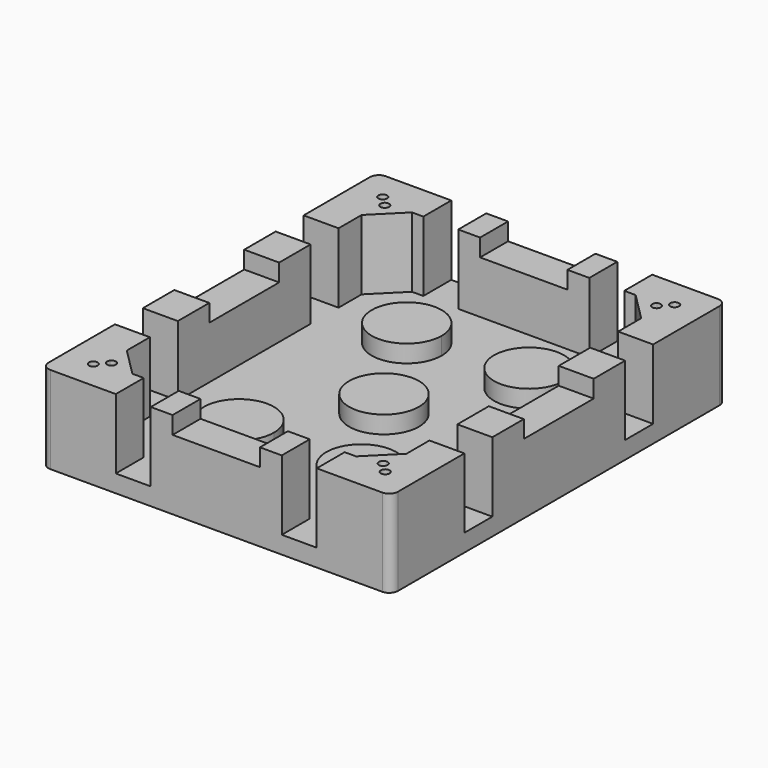
from build123d import *

# Parameters (mm, degrees)
F0_R     = 12.7
F0_R_2   = 1.5875
F0_W     = 6.35
F0_H     = 31.75
F0_W_2   = 31.75
F0_H_2   = 6.35
F0_H_3   = 14.2875
F0_H_4   = 12.7
F0_W_3   = 12.7
F0_W_4   = 7.9375
F1_DEPTH = 6.35
F2_DEPTH = 12.7
F3_DEPTH = 31.75
F4_DEPTH = 25.4


# Not quite as in the source:
# - a feature names something its author has since deleted; it is built from what else it names


with BuildPart() as f1:
    # F0 (on Top) → F1 (new body)
    with BuildSketch(Plane.XY):
        Polygon((-23.8125, 63.5), (-36.5125, 63.5), (-40.64, 63.5), (-50.8, 53.34), (-50.8, 42.8625), (-50.8, 30.1625), (-50.8, 15.875), (-50.8, -15.875), (-50.8, -30.1625), (-50.8, -42.8625), (-50.8, -53.34), (-40.64, -63.5), (-36.5125, -63.5), (-23.8125, -63.5), (-15.875, -63.5), (15.875, -63.5), (23.8125, -63.5), (36.5125, -63.5), (40.64, -63.5), (50.8, -53.34), (50.8, -42.8625), (50.8, -30.1625), (50.8, -15.875), (50.8, 15.875), (50.8, 30.1625), (50.8, 42.8625), (50.8, 53.34), (40.64, 63.5), (36.5125, 63.5), (23.8125, 63.5), (15.875, 63.5), (-15.875, 63.5), align=None)
        Polygon((-34.925, 38.1), (-34.925, 50.8), (-22.225, 50.8), (22.2250000973, 50.8), (34.925, 50.8), (34.925, 38.1), (34.925, -38.1), (34.925, -50.8), (22.2249999213, -50.8), (-22.225, -50.8), (-34.925, -50.8), (-34.925, -38.1), align=None, mode=Mode.SUBTRACT)
        with BuildLine():
            Line((22.2250000973, 50.8), (-22.225, 50.8))
            ThreePointArc((-22.225, 50.8), (-13.2447438789, 47.0802561211), (-9.525, 38.1))
            ThreePointArc((-9.525, 38.1), (-22.225, 25.4), (-34.925, 38.1))
            Line((-34.925, 38.1), (-34.925, -38.1))
            ThreePointArc((-34.925, -38.1), (-22.225, -25.4), (-9.525, -38.1))
            ThreePointArc((-9.525, -38.1), (-13.2447438789, -47.0802561211), (-22.225, -50.8))
            Line((-22.225, -50.8), (22.2249999213, -50.8))
            ThreePointArc((22.2249999213, -50.8), (13.2447439068, -29.1197438511), (34.925, -38.1))
            Line((34.925, -38.1), (34.925, 38.1))
            ThreePointArc((34.925, 38.1), (13.2447438445, 29.1197439133), (22.2250000973, 50.8))
        make_face()
        Circle(F0_R, mode=Mode.SUBTRACT)
        with BuildLine():
            ThreePointArc((34.925, 38.1), (31.2052561555, 47.0802560867), (22.2250000973, 50.8))
            ThreePointArc((22.2250000973, 50.8), (13.2447438445, 29.1197439133), (34.925, 38.1))
        make_face()
        Circle(F0_R)
        with BuildLine():
            ThreePointArc((-9.525, -38.1), (-22.225, -25.4), (-34.925, -38.1))
            ThreePointArc((-34.925, -38.1), (-31.2052561211, -47.0802561211), (-22.225, -50.8))
            ThreePointArc((-22.225, -50.8), (-13.2447438789, -47.0802561211), (-9.525, -38.1))
        make_face()
        with BuildLine():
            ThreePointArc((22.2249999213, -50.8), (31.2052560932, -47.0802561489), (34.925, -38.1))
            ThreePointArc((34.925, -38.1), (13.2447439068, -29.1197438511), (22.2249999213, -50.8))
        make_face()
        with BuildLine():
            ThreePointArc((-9.525, 38.1), (-13.2447438789, 47.0802561211), (-22.225, 50.8))
            ThreePointArc((-22.225, 50.8), (-31.2052561211, 47.0802561211), (-34.925, 38.1))
            ThreePointArc((-34.925, 38.1), (-22.225, 25.4), (-9.525, 38.1))
        make_face()
        with BuildLine():
            Line((-57.15, -42.8625), (-63.5, -42.8625))
            Line((-63.5, -42.8625), (-63.5, -73.025))
            ThreePointArc((-63.5, -73.025), (-62.5700640303, -75.2700640303), (-60.325, -76.2))
            Line((-60.325, -76.2), (-36.5125, -76.2))
            Line((-36.5125, -76.2), (-36.5125, -69.85))
            Line((-36.5125, -69.85), (-53.975, -69.85))
            ThreePointArc((-53.975, -69.85), (-56.2200640303, -68.9200640303), (-57.15, -66.675))
            Line((-57.15, -66.675), (-57.15, -42.8625))
        make_face()
        with BuildLine():
            Line((-36.5125, 76.2), (-60.325, 76.2))
            ThreePointArc((-60.325, 76.2), (-62.5700640303, 75.2700640303), (-63.5, 73.025))
            Line((-63.5, 73.025), (-63.5, 42.8625))
            Line((-63.5, 42.8625), (-57.15, 42.8625))
            Line((-57.15, 42.8625), (-57.15, 66.675))
            ThreePointArc((-57.15, 66.675), (-56.2200640303, 68.9200640303), (-53.975, 69.85))
            Line((-53.975, 69.85), (-36.5125, 69.85))
            Line((-36.5125, 69.85), (-36.5125, 76.2))
        make_face()
        with BuildLine():
            Line((60.325, 76.2), (36.5125, 76.2))
            Line((36.5125, 76.2), (36.5125, 69.85))
            Line((36.5125, 69.85), (53.975, 69.85))
            ThreePointArc((53.975, 69.85), (56.2200640303, 68.9200640303), (57.15, 66.675))
            Line((57.15, 66.675), (57.15, 42.8625))
            Line((57.15, 42.8625), (63.5, 42.8625))
            Line((63.5, 42.8625), (63.5, 73.025))
            ThreePointArc((63.5, 73.025), (62.5700640303, 75.2700640303), (60.325, 76.2))
        make_face()
        with BuildLine():
            Line((63.5, -73.025), (63.5, -42.8625))
            Line((63.5, -42.8625), (57.15, -42.8625))
            Line((57.15, -42.8625), (57.15, -66.675))
            ThreePointArc((57.15, -66.675), (56.2200640303, -68.9200640303), (53.975, -69.85))
            Line((53.975, -69.85), (36.5125, -69.85))
            Line((36.5125, -69.85), (36.5125, -76.2))
            Line((36.5125, -76.2), (60.325, -76.2))
            ThreePointArc((60.325, -76.2), (62.5700640303, -75.2700640303), (63.5, -73.025))
        make_face()
        with BuildLine():
            Line((-50.8, -42.8625), (-57.15, -42.8625))
            Line((-57.15, -42.8625), (-57.15, -66.675))
            ThreePointArc((-57.15, -66.675), (-56.2200640303, -68.9200640303), (-53.975, -69.85))
            Line((-53.975, -69.85), (-36.5125, -69.85))
            Line((-36.5125, -69.85), (-36.5125, -63.5))
            Line((-36.5125, -63.5), (-40.64, -63.5))
            Line((-40.64, -63.5), (-47.625, -63.5))
            ThreePointArc((-47.625, -63.5), (-48.054315115, -63.4708406718), (-48.4757445352, -63.3838982879))
            ThreePointArc((-48.4757445352, -63.3838982879), (-50.4996408811, -63.1996408811), (-50.6838982879, -61.1757445352))
            ThreePointArc((-50.6838982879, -61.1757445352), (-50.7708406718, -60.754315115), (-50.8, -60.325))
            Line((-50.8, -60.325), (-50.8, -53.34))
            Line((-50.8, -53.34), (-50.8, -42.8625))
        make_face()
        with Locations((-53.0410533634, -65.7410533634)):
            Circle(F0_R_2, mode=Mode.SUBTRACT)
        with BuildLine():
            Line((53.975, 69.85), (36.5125, 69.85))
            Line((36.5125, 69.85), (36.5125, 63.5))
            Line((36.5125, 63.5), (40.64, 63.5))
            Line((40.64, 63.5), (47.625, 63.5))
            ThreePointArc((47.625, 63.5), (48.054315115, 63.4708406718), (48.4757445352, 63.3838982879))
            ThreePointArc((48.4757445352, 63.3838982879), (50.1150927327, 63.4826465078), (50.964608866, 62.077108866))
            ThreePointArc((50.964608866, 62.077108866), (50.8928074603, 61.6050770648), (50.6838982879, 61.1757445352))
            ThreePointArc((50.6838982879, 61.1757445352), (50.7708406718, 60.754315115), (50.8, 60.325))
            Line((50.8, 60.325), (50.8, 53.34))
            Line((50.8, 53.34), (50.8, 42.8625))
            Line((50.8, 42.8625), (57.15, 42.8625))
            Line((57.15, 42.8625), (57.15, 66.675))
            ThreePointArc((57.15, 66.675), (56.2200640303, 68.9200640303), (53.975, 69.85))
        make_face()
        with Locations((53.0410533634, 65.7410533634)):
            Circle(F0_R_2, mode=Mode.SUBTRACT)
        with BuildLine():
            Line((-36.5125, 63.5), (-36.5125, 69.85))
            Line((-36.5125, 69.85), (-53.975, 69.85))
            ThreePointArc((-53.975, 69.85), (-56.2200640303, 68.9200640303), (-57.15, 66.675))
            Line((-57.15, 66.675), (-57.15, 42.8625))
            Line((-57.15, 42.8625), (-50.8, 42.8625))
            Line((-50.8, 42.8625), (-50.8, 53.34))
            Line((-50.8, 53.34), (-50.8, 60.325))
            ThreePointArc((-50.8, 60.325), (-50.7708406718, 60.754315115), (-50.6838982879, 61.1757445352))
            ThreePointArc((-50.6838982879, 61.1757445352), (-50.4996408811, 63.1996408811), (-48.4757445352, 63.3838982879))
            ThreePointArc((-48.4757445352, 63.3838982879), (-48.054315115, 63.4708406718), (-47.625, 63.5))
            Line((-47.625, 63.5), (-40.64, 63.5))
            Line((-40.64, 63.5), (-36.5125, 63.5))
        make_face()
        with Locations((-53.0410533634, 65.7410533634)):
            Circle(F0_R_2, mode=Mode.SUBTRACT)
        with BuildLine():
            Line((57.15, -66.675), (57.15, -42.8625))
            Line((57.15, -42.8625), (50.8, -42.8625))
            Line((50.8, -42.8625), (50.8, -53.34))
            Line((50.8, -53.34), (50.8, -60.9545768509))
            ThreePointArc((50.8, -60.9545768509), (50.7933363337, -61.1386401459), (50.7733802244, -61.3217397219))
            ThreePointArc((50.7733802244, -61.3217397219), (50.9160593252, -61.6875094123), (50.964608866, -62.077108866))
            ThreePointArc((50.964608866, -62.077108866), (50.1898227559, -63.4407995872), (48.6217397219, -63.4733802244))
            ThreePointArc((48.6217397219, -63.4733802244), (48.4386401459, -63.4933363337), (48.2545768509, -63.5))
            Line((48.2545768509, -63.5), (40.64, -63.5))
            Line((40.64, -63.5), (36.5125, -63.5))
            Line((36.5125, -63.5), (36.5125, -69.85))
            Line((36.5125, -69.85), (53.975, -69.85))
            ThreePointArc((53.975, -69.85), (56.2200640303, -68.9200640303), (57.15, -66.675))
        make_face()
        with Locations((53.0410533634, -65.7410533634)):
            Circle(F0_R_2, mode=Mode.SUBTRACT)
        with Locations((-60.325, 0)):
            Rectangle(F0_W, F0_H)
        with Locations((0, -73.025)):
            Rectangle(F0_W_2, F0_H_2)
        with Locations((0, 66.675)):
            Rectangle(F0_W_2, F0_H_2)
        with Locations((0, 73.025)):
            Rectangle(F0_W_2, F0_H_2)
        with Locations((-53.975, 0)):
            Rectangle(F0_W, F0_H)
        with Locations((53.975, 0)):
            Rectangle(F0_W, F0_H)
        with Locations((0, -66.675)):
            Rectangle(F0_W_2, F0_H_2)
        with Locations((60.325, 0)):
            Rectangle(F0_W, F0_H)
        with Locations((60.325, -23.01875)):
            Rectangle(F0_W, F0_H_3)
        with Locations((-53.975, -23.01875)):
            Rectangle(F0_W, F0_H_3)
        with Locations((-53.975, 23.01875)):
            Rectangle(F0_W, F0_H_3)
        with Locations((53.975, -23.01875)):
            Rectangle(F0_W, F0_H_3)
        with Locations((53.975, 23.01875)):
            Rectangle(F0_W, F0_H_3)
        with Locations((-60.325, -23.01875)):
            Rectangle(F0_W, F0_H_3)
        with Locations((60.325, 23.01875)):
            Rectangle(F0_W, F0_H_3)
        with Locations((-60.325, 23.01875)):
            Rectangle(F0_W, F0_H_3)
        with Locations((-60.325, -36.5125)):
            Rectangle(F0_W, F0_H_4)
        with Locations((53.975, 36.5125)):
            Rectangle(F0_W, F0_H_4)
        with Locations((30.1625, 73.025)):
            Rectangle(F0_W_3, F0_H_2)
        with Locations((60.325, -36.5125)):
            Rectangle(F0_W, F0_H_4)
        with Locations((60.325, 36.5125)):
            Rectangle(F0_W, F0_H_4)
        with Locations((-60.325, 36.5125)):
            Rectangle(F0_W, F0_H_4)
        with Locations((-30.1625, -73.025)):
            Rectangle(F0_W_3, F0_H_2)
        with Locations((30.1625, -66.675)):
            Rectangle(F0_W_3, F0_H_2)
        with Locations((30.1625, -73.025)):
            Rectangle(F0_W_3, F0_H_2)
        with Locations((-30.1625, 73.025)):
            Rectangle(F0_W_3, F0_H_2)
        with Locations((-30.1625, -66.675)):
            Rectangle(F0_W_3, F0_H_2)
        with Locations((-53.975, -36.5125)):
            Rectangle(F0_W, F0_H_4)
        with Locations((-53.975, 36.5125)):
            Rectangle(F0_W, F0_H_4)
        with Locations((-30.1625, 66.675)):
            Rectangle(F0_W_3, F0_H_2)
        with Locations((53.975, -36.5125)):
            Rectangle(F0_W, F0_H_4)
        with Locations((30.1625, 66.675)):
            Rectangle(F0_W_3, F0_H_2)
        with Locations((19.84375, -66.675)):
            Rectangle(F0_W_4, F0_H_2)
        with Locations((-19.84375, -66.675)):
            Rectangle(F0_W_4, F0_H_2)
        with Locations((19.84375, 73.025)):
            Rectangle(F0_W_4, F0_H_2)
        with Locations((-19.84375, 73.025)):
            Rectangle(F0_W_4, F0_H_2)
        with Locations((-19.84375, 66.675)):
            Rectangle(F0_W_4, F0_H_2)
        with Locations((-19.84375, -73.025)):
            Rectangle(F0_W_4, F0_H_2)
        with Locations((19.84375, -73.025)):
            Rectangle(F0_W_4, F0_H_2)
        with Locations((19.84375, 66.675)):
            Rectangle(F0_W_4, F0_H_2)
        with BuildLine():
            Line((50.8, -60.9545768509), (50.8, -53.34))
            Line((50.8, -53.34), (40.64, -63.5))
            Line((40.64, -63.5), (48.2545768509, -63.5))
            ThreePointArc((48.2545768509, -63.5), (48.4386401459, -63.4933363337), (48.6217397219, -63.4733802244))
            ThreePointArc((48.6217397219, -63.4733802244), (48.2545768509, -60.9545768509), (50.7733802244, -61.3217397219))
            ThreePointArc((50.7733802244, -61.3217397219), (50.7933363337, -61.1386401459), (50.8, -60.9545768509))
        make_face()
        with BuildLine():
            Line((-50.8, 53.34), (-40.64, 63.5))
            Line((-40.64, 63.5), (-47.625, 63.5))
            ThreePointArc((-47.625, 63.5), (-48.054315115, 63.4708406718), (-48.4757445352, 63.3838982879))
            ThreePointArc((-48.4757445352, 63.3838982879), (-47.9715712242, 62.8150927327), (-47.789608866, 62.077108866))
            ThreePointArc((-47.789608866, 62.077108866), (-48.9050770648, 60.5614102718), (-50.6838982879, 61.1757445352))
            ThreePointArc((-50.6838982879, 61.1757445352), (-50.7708406718, 60.754315115), (-50.8, 60.325))
            Line((-50.8, 60.325), (-50.8, 53.34))
        make_face()
        with BuildLine():
            Line((-40.64, -63.5), (-50.8, -53.34))
            Line((-50.8, -53.34), (-50.8, -60.325))
            ThreePointArc((-50.8, -60.325), (-50.7708406718, -60.754315115), (-50.6838982879, -61.1757445352))
            ThreePointArc((-50.6838982879, -61.1757445352), (-48.9050770648, -60.5614102718), (-47.789608866, -62.077108866))
            ThreePointArc((-47.789608866, -62.077108866), (-47.9715712242, -62.8150927327), (-48.4757445352, -63.3838982879))
            ThreePointArc((-48.4757445352, -63.3838982879), (-48.054315115, -63.4708406718), (-47.625, -63.5))
            Line((-47.625, -63.5), (-40.64, -63.5))
        make_face()
        with BuildLine():
            Line((47.625, 63.5), (40.64, 63.5))
            Line((40.64, 63.5), (50.8, 53.34))
            Line((50.8, 53.34), (50.8, 60.325))
            ThreePointArc((50.8, 60.325), (50.7708406718, 60.754315115), (50.6838982879, 61.1757445352))
            ThreePointArc((50.6838982879, 61.1757445352), (48.2545768509, 60.9545768509), (48.4757445352, 63.3838982879))
            ThreePointArc((48.4757445352, 63.3838982879), (48.054315115, 63.4708406718), (47.625, 63.5))
        make_face()
        with BuildLine():
            Line((34.925, 50.8), (22.2250000973, 50.8))
            ThreePointArc((22.2250000973, 50.8), (31.2052561555, 47.0802560867), (34.925, 38.1))
            Line((34.925, 38.1), (34.925, 50.8))
        make_face()
        with BuildLine():
            Line((34.925, -50.8), (34.925, -38.1))
            ThreePointArc((34.925, -38.1), (31.2052560932, -47.0802561489), (22.2249999213, -50.8))
            Line((22.2249999213, -50.8), (34.925, -50.8))
        make_face()
        with BuildLine():
            ThreePointArc((-22.225, -50.8), (-31.2052561211, -47.0802561211), (-34.925, -38.1))
            Line((-34.925, -38.1), (-34.925, -50.8))
            Line((-34.925, -50.8), (-22.225, -50.8))
        make_face()
        with BuildLine():
            Line((-22.225, 50.8), (-34.925, 50.8))
            Line((-34.925, 50.8), (-34.925, 38.1))
            ThreePointArc((-34.925, 38.1), (-31.2052561211, 47.0802561211), (-22.225, 50.8))
        make_face()
        with Locations((-53.0410533634, 65.7410533634)):
            Circle(F0_R_2)
        with Locations((53.0410533634, 65.7410533634)):
            Circle(F0_R_2)
        with Locations((53.0410533634, -65.7410533634)):
            Circle(F0_R_2)
        with Locations((-53.0410533634, -65.7410533634)):
            Circle(F0_R_2)
        with BuildLine():
            ThreePointArc((48.6217397219, -63.4733802244), (50.0544628206, -62.7544628206), (50.7733802244, -61.3217397219))
            ThreePointArc((50.7733802244, -61.3217397219), (48.2545768509, -60.9545768509), (48.6217397219, -63.4733802244))
        make_face()
        with BuildLine():
            ThreePointArc((-47.789608866, 62.077108866), (-47.9715712242, 62.8150927327), (-48.4757445352, 63.3838982879))
            ThreePointArc((-48.4757445352, 63.3838982879), (-49.8700640303, 62.5700640303), (-50.6838982879, 61.1757445352))
            ThreePointArc((-50.6838982879, 61.1757445352), (-48.9050770648, 60.5614102718), (-47.789608866, 62.077108866))
        make_face()
        with BuildLine():
            ThreePointArc((50.6838982879, 61.1757445352), (49.8700640303, 62.5700640303), (48.4757445352, 63.3838982879))
            ThreePointArc((48.4757445352, 63.3838982879), (48.2545768509, 60.9545768509), (50.6838982879, 61.1757445352))
        make_face()
        with BuildLine():
            ThreePointArc((-47.789608866, -62.077108866), (-48.9050770648, -60.5614102718), (-50.6838982879, -61.1757445352))
            ThreePointArc((-50.6838982879, -61.1757445352), (-49.8700640303, -62.5700640303), (-48.4757445352, -63.3838982879))
            ThreePointArc((-48.4757445352, -63.3838982879), (-47.9715712242, -62.8150927327), (-47.789608866, -62.077108866))
        make_face()
        with BuildLine():
            ThreePointArc((50.964608866, 62.077108866), (50.1150927327, 63.4826465078), (48.4757445352, 63.3838982879))
            ThreePointArc((48.4757445352, 63.3838982879), (49.8700640303, 62.5700640303), (50.6838982879, 61.1757445352))
            ThreePointArc((50.6838982879, 61.1757445352), (50.8928074603, 61.6050770648), (50.964608866, 62.077108866))
        make_face()
        with BuildLine():
            ThreePointArc((-50.6838982879, 61.1757445352), (-49.8700640303, 62.5700640303), (-48.4757445352, 63.3838982879))
            ThreePointArc((-48.4757445352, 63.3838982879), (-50.4996408811, 63.1996408811), (-50.6838982879, 61.1757445352))
        make_face()
        with BuildLine():
            ThreePointArc((-48.4757445352, -63.3838982879), (-49.8700640303, -62.5700640303), (-50.6838982879, -61.1757445352))
            ThreePointArc((-50.6838982879, -61.1757445352), (-50.4996408811, -63.1996408811), (-48.4757445352, -63.3838982879))
        make_face()
        with BuildLine():
            ThreePointArc((50.964608866, -62.077108866), (50.9160593252, -61.6875094123), (50.7733802244, -61.3217397219))
            ThreePointArc((50.7733802244, -61.3217397219), (50.0544628206, -62.7544628206), (48.6217397219, -63.4733802244))
            ThreePointArc((48.6217397219, -63.4733802244), (50.1898227559, -63.4407995872), (50.964608866, -62.077108866))
        make_face()
    extrude(amount=F1_DEPTH)

    # F0 (on Top) → F2 (join)
    with BuildSketch(Plane.XY):
        with BuildLine():
            ThreePointArc((-9.525, 38.1), (-13.2447438789, 47.0802561211), (-22.225, 50.8))
            ThreePointArc((-22.225, 50.8), (-31.2052561211, 47.0802561211), (-34.925, 38.1))
            ThreePointArc((-34.925, 38.1), (-22.225, 25.4), (-9.525, 38.1))
        make_face()
        with BuildLine():
            ThreePointArc((34.925, 38.1), (31.2052561555, 47.0802560867), (22.2250000973, 50.8))
            ThreePointArc((22.2250000973, 50.8), (13.2447438445, 29.1197439133), (34.925, 38.1))
        make_face()
        Circle(F0_R)
        with BuildLine():
            ThreePointArc((-9.525, -38.1), (-22.225, -25.4), (-34.925, -38.1))
            ThreePointArc((-34.925, -38.1), (-31.2052561211, -47.0802561211), (-22.225, -50.8))
            ThreePointArc((-22.225, -50.8), (-13.2447438789, -47.0802561211), (-9.525, -38.1))
        make_face()
        with BuildLine():
            ThreePointArc((22.2249999213, -50.8), (31.2052560932, -47.0802561489), (34.925, -38.1))
            ThreePointArc((34.925, -38.1), (13.2447439068, -29.1197438511), (22.2249999213, -50.8))
        make_face()
    extrude(amount=F2_DEPTH)

    # F0 (on Top) → F3 (join)
    with BuildSketch(Plane.XY):
        with BuildLine():
            Line((-36.5125, 76.2), (-60.325, 76.2))
            ThreePointArc((-60.325, 76.2), (-62.5700640303, 75.2700640303), (-63.5, 73.025))
            Line((-63.5, 73.025), (-63.5, 42.8625))
            Line((-63.5, 42.8625), (-57.15, 42.8625))
            Line((-57.15, 42.8625), (-57.15, 66.675))
            ThreePointArc((-57.15, 66.675), (-56.2200640303, 68.9200640303), (-53.975, 69.85))
            Line((-53.975, 69.85), (-36.5125, 69.85))
            Line((-36.5125, 69.85), (-36.5125, 76.2))
        make_face()
        with BuildLine():
            Line((-36.5125, 63.5), (-36.5125, 69.85))
            Line((-36.5125, 69.85), (-53.975, 69.85))
            ThreePointArc((-53.975, 69.85), (-56.2200640303, 68.9200640303), (-57.15, 66.675))
            Line((-57.15, 66.675), (-57.15, 42.8625))
            Line((-57.15, 42.8625), (-50.8, 42.8625))
            Line((-50.8, 42.8625), (-50.8, 53.34))
            Line((-50.8, 53.34), (-50.8, 60.325))
            ThreePointArc((-50.8, 60.325), (-50.7708406718, 60.754315115), (-50.6838982879, 61.1757445352))
            ThreePointArc((-50.6838982879, 61.1757445352), (-50.4996408811, 63.1996408811), (-48.4757445352, 63.3838982879))
            ThreePointArc((-48.4757445352, 63.3838982879), (-48.054315115, 63.4708406718), (-47.625, 63.5))
            Line((-47.625, 63.5), (-40.64, 63.5))
            Line((-40.64, 63.5), (-36.5125, 63.5))
        make_face()
        with Locations((-53.0410533634, 65.7410533634)):
            Circle(F0_R_2, mode=Mode.SUBTRACT)
        with Locations((-19.84375, 73.025)):
            Rectangle(F0_W_4, F0_H_2)
        with Locations((-19.84375, 66.675)):
            Rectangle(F0_W_4, F0_H_2)
        with BuildLine():
            Line((-50.8, 53.34), (-40.64, 63.5))
            Line((-40.64, 63.5), (-47.625, 63.5))
            ThreePointArc((-47.625, 63.5), (-48.054315115, 63.4708406718), (-48.4757445352, 63.3838982879))
            ThreePointArc((-48.4757445352, 63.3838982879), (-47.9715712242, 62.8150927327), (-47.789608866, 62.077108866))
            ThreePointArc((-47.789608866, 62.077108866), (-48.9050770648, 60.5614102718), (-50.6838982879, 61.1757445352))
            ThreePointArc((-50.6838982879, 61.1757445352), (-50.7708406718, 60.754315115), (-50.8, 60.325))
            Line((-50.8, 60.325), (-50.8, 53.34))
        make_face()
        with Locations((19.84375, 73.025)):
            Rectangle(F0_W_4, F0_H_2)
        with Locations((19.84375, 66.675)):
            Rectangle(F0_W_4, F0_H_2)
        with BuildLine():
            Line((60.325, 76.2), (36.5125, 76.2))
            Line((36.5125, 76.2), (36.5125, 69.85))
            Line((36.5125, 69.85), (53.975, 69.85))
            ThreePointArc((53.975, 69.85), (56.2200640303, 68.9200640303), (57.15, 66.675))
            Line((57.15, 66.675), (57.15, 42.8625))
            Line((57.15, 42.8625), (63.5, 42.8625))
            Line((63.5, 42.8625), (63.5, 73.025))
            ThreePointArc((63.5, 73.025), (62.5700640303, 75.2700640303), (60.325, 76.2))
        make_face()
        with BuildLine():
            Line((53.975, 69.85), (36.5125, 69.85))
            Line((36.5125, 69.85), (36.5125, 63.5))
            Line((36.5125, 63.5), (40.64, 63.5))
            Line((40.64, 63.5), (47.625, 63.5))
            ThreePointArc((47.625, 63.5), (48.054315115, 63.4708406718), (48.4757445352, 63.3838982879))
            ThreePointArc((48.4757445352, 63.3838982879), (50.1150927327, 63.4826465078), (50.964608866, 62.077108866))
            ThreePointArc((50.964608866, 62.077108866), (50.8928074603, 61.6050770648), (50.6838982879, 61.1757445352))
            ThreePointArc((50.6838982879, 61.1757445352), (50.7708406718, 60.754315115), (50.8, 60.325))
            Line((50.8, 60.325), (50.8, 53.34))
            Line((50.8, 53.34), (50.8, 42.8625))
            Line((50.8, 42.8625), (57.15, 42.8625))
            Line((57.15, 42.8625), (57.15, 66.675))
            ThreePointArc((57.15, 66.675), (56.2200640303, 68.9200640303), (53.975, 69.85))
        make_face()
        with Locations((53.0410533634, 65.7410533634)):
            Circle(F0_R_2, mode=Mode.SUBTRACT)
        with BuildLine():
            Line((47.625, 63.5), (40.64, 63.5))
            Line((40.64, 63.5), (50.8, 53.34))
            Line((50.8, 53.34), (50.8, 60.325))
            ThreePointArc((50.8, 60.325), (50.7708406718, 60.754315115), (50.6838982879, 61.1757445352))
            ThreePointArc((50.6838982879, 61.1757445352), (48.2545768509, 60.9545768509), (48.4757445352, 63.3838982879))
            ThreePointArc((48.4757445352, 63.3838982879), (48.054315115, 63.4708406718), (47.625, 63.5))
        make_face()
        with Locations((-60.325, 23.01875)):
            Rectangle(F0_W, F0_H_3)
        with Locations((-53.975, 23.01875)):
            Rectangle(F0_W, F0_H_3)
        with Locations((53.975, 23.01875)):
            Rectangle(F0_W, F0_H_3)
        with Locations((60.325, 23.01875)):
            Rectangle(F0_W, F0_H_3)
        with Locations((60.325, -23.01875)):
            Rectangle(F0_W, F0_H_3)
        with Locations((53.975, -23.01875)):
            Rectangle(F0_W, F0_H_3)
        with Locations((-53.975, -23.01875)):
            Rectangle(F0_W, F0_H_3)
        with Locations((-60.325, -23.01875)):
            Rectangle(F0_W, F0_H_3)
        with BuildLine():
            Line((-57.15, -42.8625), (-63.5, -42.8625))
            Line((-63.5, -42.8625), (-63.5, -73.025))
            ThreePointArc((-63.5, -73.025), (-62.5700640303, -75.2700640303), (-60.325, -76.2))
            Line((-60.325, -76.2), (-36.5125, -76.2))
            Line((-36.5125, -76.2), (-36.5125, -69.85))
            Line((-36.5125, -69.85), (-53.975, -69.85))
            ThreePointArc((-53.975, -69.85), (-56.2200640303, -68.9200640303), (-57.15, -66.675))
            Line((-57.15, -66.675), (-57.15, -42.8625))
        make_face()
        with BuildLine():
            Line((-50.8, -42.8625), (-57.15, -42.8625))
            Line((-57.15, -42.8625), (-57.15, -66.675))
            ThreePointArc((-57.15, -66.675), (-56.2200640303, -68.9200640303), (-53.975, -69.85))
            Line((-53.975, -69.85), (-36.5125, -69.85))
            Line((-36.5125, -69.85), (-36.5125, -63.5))
            Line((-36.5125, -63.5), (-40.64, -63.5))
            Line((-40.64, -63.5), (-47.625, -63.5))
            ThreePointArc((-47.625, -63.5), (-48.054315115, -63.4708406718), (-48.4757445352, -63.3838982879))
            ThreePointArc((-48.4757445352, -63.3838982879), (-50.4996408811, -63.1996408811), (-50.6838982879, -61.1757445352))
            ThreePointArc((-50.6838982879, -61.1757445352), (-50.7708406718, -60.754315115), (-50.8, -60.325))
            Line((-50.8, -60.325), (-50.8, -53.34))
            Line((-50.8, -53.34), (-50.8, -42.8625))
        make_face()
        with Locations((-53.0410533634, -65.7410533634)):
            Circle(F0_R_2, mode=Mode.SUBTRACT)
        with BuildLine():
            Line((-40.64, -63.5), (-50.8, -53.34))
            Line((-50.8, -53.34), (-50.8, -60.325))
            ThreePointArc((-50.8, -60.325), (-50.7708406718, -60.754315115), (-50.6838982879, -61.1757445352))
            ThreePointArc((-50.6838982879, -61.1757445352), (-48.9050770648, -60.5614102718), (-47.789608866, -62.077108866))
            ThreePointArc((-47.789608866, -62.077108866), (-47.9715712242, -62.8150927327), (-48.4757445352, -63.3838982879))
            ThreePointArc((-48.4757445352, -63.3838982879), (-48.054315115, -63.4708406718), (-47.625, -63.5))
            Line((-47.625, -63.5), (-40.64, -63.5))
        make_face()
        with BuildLine():
            Line((50.8, -60.9545768509), (50.8, -53.34))
            Line((50.8, -53.34), (40.64, -63.5))
            Line((40.64, -63.5), (48.2545768509, -63.5))
            ThreePointArc((48.2545768509, -63.5), (48.4386401459, -63.4933363337), (48.6217397219, -63.4733802244))
            ThreePointArc((48.6217397219, -63.4733802244), (48.2545768509, -60.9545768509), (50.7733802244, -61.3217397219))
            ThreePointArc((50.7733802244, -61.3217397219), (50.7933363337, -61.1386401459), (50.8, -60.9545768509))
        make_face()
        with BuildLine():
            Line((57.15, -66.675), (57.15, -42.8625))
            Line((57.15, -42.8625), (50.8, -42.8625))
            Line((50.8, -42.8625), (50.8, -53.34))
            Line((50.8, -53.34), (50.8, -60.9545768509))
            ThreePointArc((50.8, -60.9545768509), (50.7933363337, -61.1386401459), (50.7733802244, -61.3217397219))
            ThreePointArc((50.7733802244, -61.3217397219), (50.9160593252, -61.6875094123), (50.964608866, -62.077108866))
            ThreePointArc((50.964608866, -62.077108866), (50.1898227559, -63.4407995872), (48.6217397219, -63.4733802244))
            ThreePointArc((48.6217397219, -63.4733802244), (48.4386401459, -63.4933363337), (48.2545768509, -63.5))
            Line((48.2545768509, -63.5), (40.64, -63.5))
            Line((40.64, -63.5), (36.5125, -63.5))
            Line((36.5125, -63.5), (36.5125, -69.85))
            Line((36.5125, -69.85), (53.975, -69.85))
            ThreePointArc((53.975, -69.85), (56.2200640303, -68.9200640303), (57.15, -66.675))
        make_face()
        with Locations((53.0410533634, -65.7410533634)):
            Circle(F0_R_2, mode=Mode.SUBTRACT)
        with BuildLine():
            Line((63.5, -73.025), (63.5, -42.8625))
            Line((63.5, -42.8625), (57.15, -42.8625))
            Line((57.15, -42.8625), (57.15, -66.675))
            ThreePointArc((57.15, -66.675), (56.2200640303, -68.9200640303), (53.975, -69.85))
            Line((53.975, -69.85), (36.5125, -69.85))
            Line((36.5125, -69.85), (36.5125, -76.2))
            Line((36.5125, -76.2), (60.325, -76.2))
            ThreePointArc((60.325, -76.2), (62.5700640303, -75.2700640303), (63.5, -73.025))
        make_face()
        with Locations((19.84375, -66.675)):
            Rectangle(F0_W_4, F0_H_2)
        with Locations((19.84375, -73.025)):
            Rectangle(F0_W_4, F0_H_2)
        with Locations((-19.84375, -73.025)):
            Rectangle(F0_W_4, F0_H_2)
        with Locations((-19.84375, -66.675)):
            Rectangle(F0_W_4, F0_H_2)
    extrude(amount=F3_DEPTH)

    # F0 (on Top) → F4 (join)
    with BuildSketch(Plane.XY):
        with Locations((0, 73.025)):
            Rectangle(F0_W_2, F0_H_2)
        with Locations((0, 66.675)):
            Rectangle(F0_W_2, F0_H_2)
        with Locations((53.975, 0)):
            Rectangle(F0_W, F0_H)
        with Locations((60.325, 0)):
            Rectangle(F0_W, F0_H)
        with Locations((-53.975, 0)):
            Rectangle(F0_W, F0_H)
        with Locations((-60.325, 0)):
            Rectangle(F0_W, F0_H)
        with Locations((0, -73.025)):
            Rectangle(F0_W_2, F0_H_2)
        with Locations((0, -66.675)):
            Rectangle(F0_W_2, F0_H_2)
    extrude(amount=F4_DEPTH)


solid = f1.part
